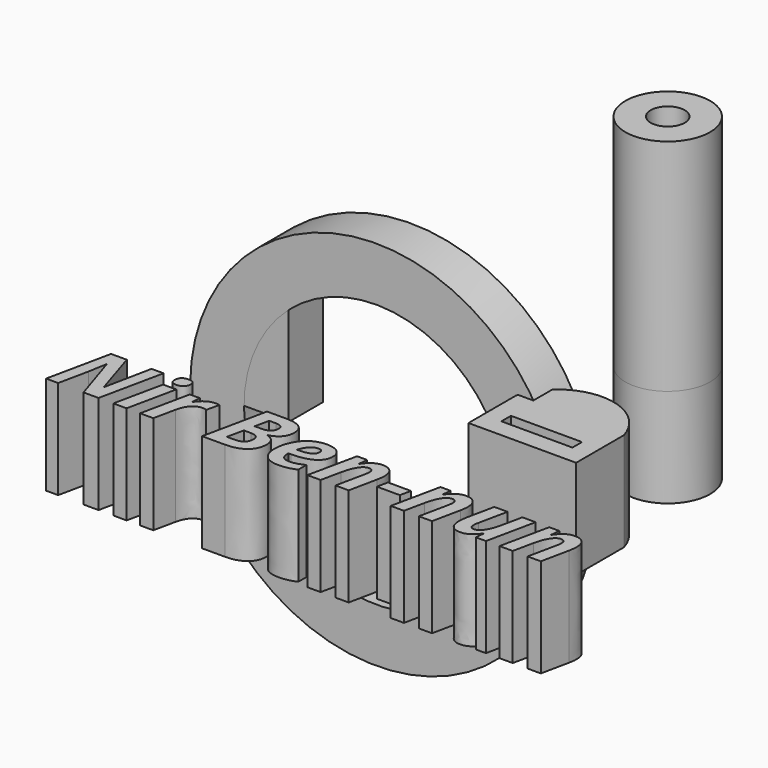
from build123d import *

# Parameters (mm, degrees)
F0_W         = 27.2673267691
F0_H         = 15.1485147695
F1_DEPTH     = 20.1
F0_R         = 10.7335211239
F0_R_2       = 4.3213563854
F2_DEPTH     = 80.7
F0_W_2       = 9
F0_H_2       = 3.0297018499
F4_DEPTH     = 25
F0_W_3       = 17.680414021
F0_H_3       = 11.0051576048
F0_TEXT_SIZE = 22.8021190398
F5_DEPTH     = 25
F5_FACE_W    = 17.680414021
F5_FACE_H    = 11.0051576048


# Not quite as in the source:
# - the program builds the solid bodies; features that only make, move or delete a surface that nothing else refers to are left out
# - Text() gives the source's letters only with a copy of the font that has no kerning and outlines rounded to 1/6400 em; it was checked with that copy


with BuildPart() as f1:
    # F0 (on Top) → F1 (new body)
    with BuildSketch(Plane.XY):
        with Locations((27.8335721353, 12.5091795269)):
            Rectangle(F0_W, F0_H)
        Polygon((18.8335721353, 12.5982882966), (27.8335721353, 12.5982882966), (36.8335721353, 12.5982882966), (36.8335721353, 9.5685864467), (27.8335721353, 9.5685864467), (18.8335721353, 9.5685864467), align=None, mode=Mode.SUBTRACT)
    extrude(amount=F1_DEPTH)

    # F0 (on Top) → F4 (cut)
    with BuildSketch(Plane.XY):
        with Locations((23.3335721353, 11.0834373716)):
            Rectangle(F0_W_2, F0_H_2)
        with Locations((32.3335721353, 11.0834373716)):
            Rectangle(F0_W_2, F0_H_2)
    extrude(amount=-F4_DEPTH, mode=Mode.SUBTRACT)


with BuildPart() as f2:
    # F0 (on Top) → F2 (new body)
    with BuildSketch(Plane.XY):
        with Locations((29.8071113217, 48.5152818465)):
            Circle(F0_R)
        with Locations((29.8071113217, 48.5152818465)):
            Circle(F0_R_2, mode=Mode.SUBTRACT)
    extrude(amount=F2_DEPTH)


with BuildPart() as f5:
    # F0 (on Top) → F5 (new body)
    with BuildSketch(Plane.XY):
        with BuildLine():
            ThreePointArc((41.4672355199, 20.0834369116), (27.8335721353, 30.2443668437), (14.1999087508, 20.0834369116))
            Line((14.1999087508, 20.0834369116), (41.4672355199, 20.0834369116))
        make_face()
        with Locations((27.8335721353, 12.5091795269)):
            Rectangle(F0_W, F0_H)
        Polygon((18.8335721353, 12.5982882966), (27.8335721353, 12.5982882966), (36.8335721353, 12.5982882966), (36.8335721353, 9.5685864467), (27.8335721353, 9.5685864467), (18.8335721353, 9.5685864467), align=None, mode=Mode.SUBTRACT)
        with Locations((29.8071113217, 48.5152818465)):
            Circle(F0_R)
        with Locations((29.8071113217, 48.5152818465)):
            Circle(F0_R_2, mode=Mode.SUBTRACT)
        with Locations((-52.6804104447, 25.9793838486)):
            Rectangle(F0_W_3, F0_H_3)
        with Locations((-63.505154103, -32.3840212077)):
            Text('Nir Ben-nun', F0_TEXT_SIZE, font='Open Sans', font_style=FontStyle.BOLDITALIC, text_align=(TextAlign.LEFT, TextAlign.BOTTOM))
    extrude(amount=F5_DEPTH)


with BuildPart() as f6:
    # F5_face (on face) → F6 (revolve)
    with BuildSketch(Plane(origin=(-52.6804104447, 25.9793838486, 25), x_dir=(1, 0, 0), z_dir=(0, 0, 1))):
        Rectangle(F5_FACE_W, F5_FACE_H)
    revolve(axis=Axis((-21.6218746298, 24.0042287586, 0), (0, -1, 0)))


solid = Compound([f1.part, f2.part, f5.part, f6.part])
